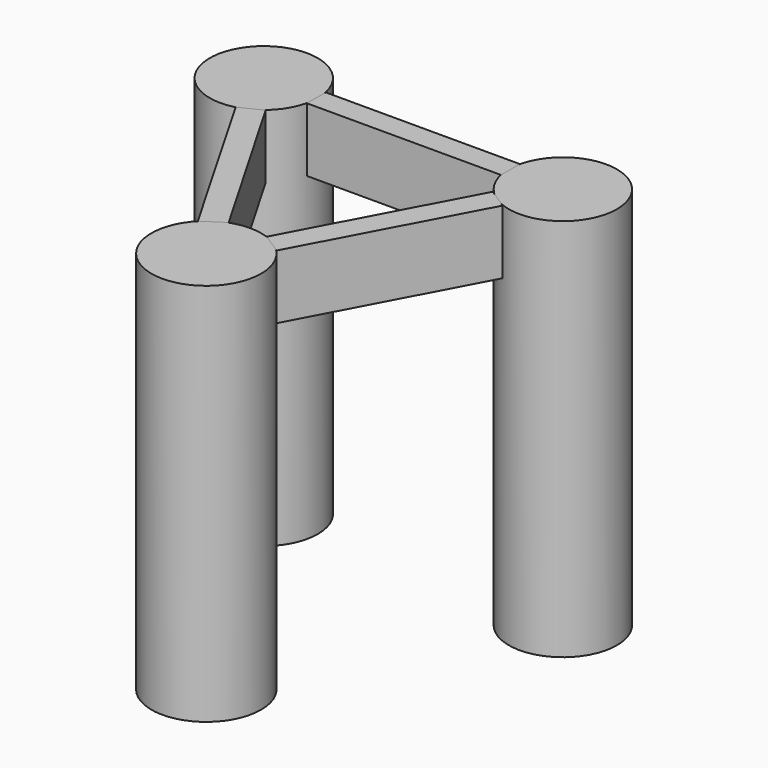
from build123d import *

# Parameters (mm, degrees)
F0_R     = 10.7297432275
F1_DEPTH = 76.2
F0_R_2   = 10.8853479612
F3_DEPTH = 12.7


# Not quite as in the source:
# - a length typed as a fraction of an inch, garbled in the dataset ("3 / 203.2 mm" for 3/8 in), is restored


with BuildPart() as f1:
    # F0 (on Top) → F1 (new body)
    with BuildSketch(Plane.XY):
        with Locations((-29.8160351813, 21.1986098439)):
            Circle(F0_R)
    extrude(amount=-F1_DEPTH)


with BuildPart() as f1b:
    # F0 (on Top) → F1, piece 2 (new body)
    with BuildSketch(Plane.XY):
        with Locations((29.6960119158, 21.0190378129)):
            Circle(F0_R)
    extrude(amount=-F1_DEPTH)


with BuildPart() as f1c:
    # F0 (on Top) → F1, piece 3 (new body)
    with BuildSketch(Plane.XY):
        with Locations((0, -30.3295161575)):
            Circle(F0_R_2)
    extrude(amount=-F1_DEPTH)


with BuildPart() as f3:
    # F2 (on Top) → F3 (new body)
    with BuildSketch(Plane.XY):
        Polygon((-19.2763544619, 23.4492365271), (-19.331432879, 18.7675692141), (19.2234721035, 18.7675692141), (19.2234721035, 23.4492365271), align=None)
    extrude(amount=-F3_DEPTH)


with BuildPart() as f3b:
    # F2 (on Top) → F3, piece 2 (new body)
    with BuildSketch(Plane.XY):
        Polygon((-27.1035581827, 10.8587807044), (-7.785834372, -22.7020327002), (-3.7693547531, -20.0526502035), (-22.8502620012, 12.9573745653), align=None)
    extrude(amount=-F3_DEPTH)


with BuildPart() as f3c:
    # F2 (on Top) → F3, piece 3 (new body)
    with BuildSketch(Plane.XY):
        Polygon((21.7406842858, 13.5751729831), (3.8015870377, -20.0973968022), (7.9187573865, -22.7441489697), (25.8416007684, 10.8979115078), align=None)
    extrude(amount=-F3_DEPTH)


solid = Compound([f1.part, f1b.part, f1c.part, f3.part, f3b.part, f3c.part])
